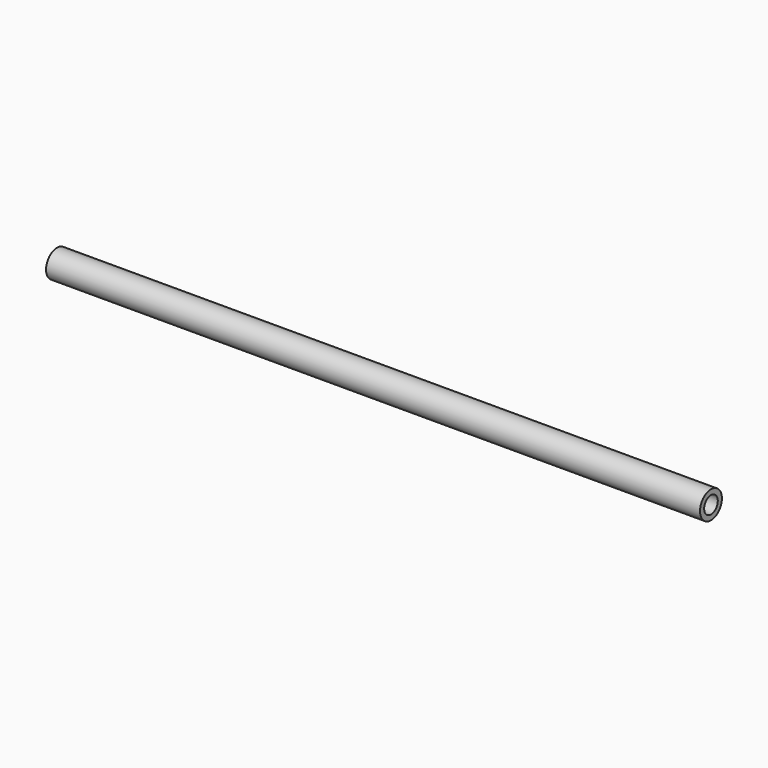
from build123d import *

# Parameters (mm, degrees)
F0_R     = 4.5
F1_DEPTH = 215
F2_R     = 2.8
F3_DEPTH = 215


with BuildPart() as f1:
    # F0 (on Right) → F1 (new body)
    with BuildSketch(Plane.YZ):
        Circle(F0_R)
    extrude(amount=F1_DEPTH)

    # F2 (on face) → F3 (cut, through all)
    with BuildSketch(Plane.YZ.offset(215)):
        Circle(F2_R)
    extrude(amount=-F3_DEPTH, mode=Mode.SUBTRACT)


solid = f1.part
